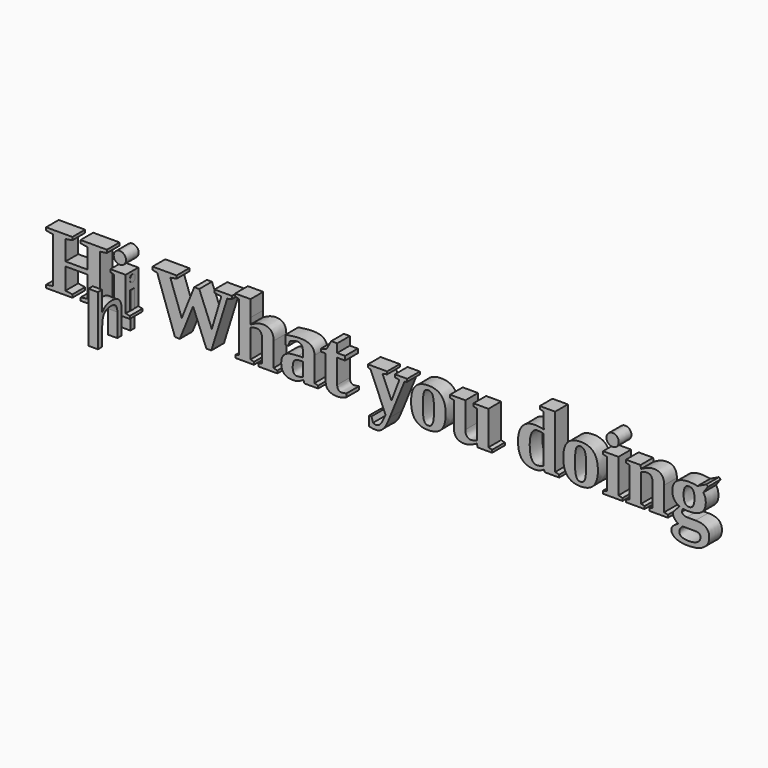
from build123d import *

# Parameters (mm, degrees)
F0_TEXT_SIZE = 65.5483894257
F1_DEPTH     = 12.7
F2_TEXT_SIZE = 53.0803265671
F3_DEPTH     = 7.62


# Not quite as in the source:
# - a feature names something its author has since deleted; it is built from what else it names
# - Text() gives the source's letters only with a copy of the font that has no kerning and outlines rounded to 1/6400 em; it was checked with that copy


with BuildPart() as f1:
    # F0 (on Front) → F1 (new body)
    with BuildSketch(Plane.XZ):
        with Locations((-57.518709451, 11.061290279)):
            Text('Hi What you doing', F0_TEXT_SIZE, font='Tinos', font_style=FontStyle.BOLD, text_align=(TextAlign.LEFT, TextAlign.BOTTOM))
    extrude(amount=F1_DEPTH)

    # F2 (on Right) → F3 (join)
    with BuildSketch(Plane.YZ):
        with Locations((-45.3007412046, 0)):
            Text('hi', F2_TEXT_SIZE, font='Open Sans', text_align=(TextAlign.LEFT, TextAlign.BOTTOM))
    extrude(amount=F3_DEPTH)


solid = f1.part
